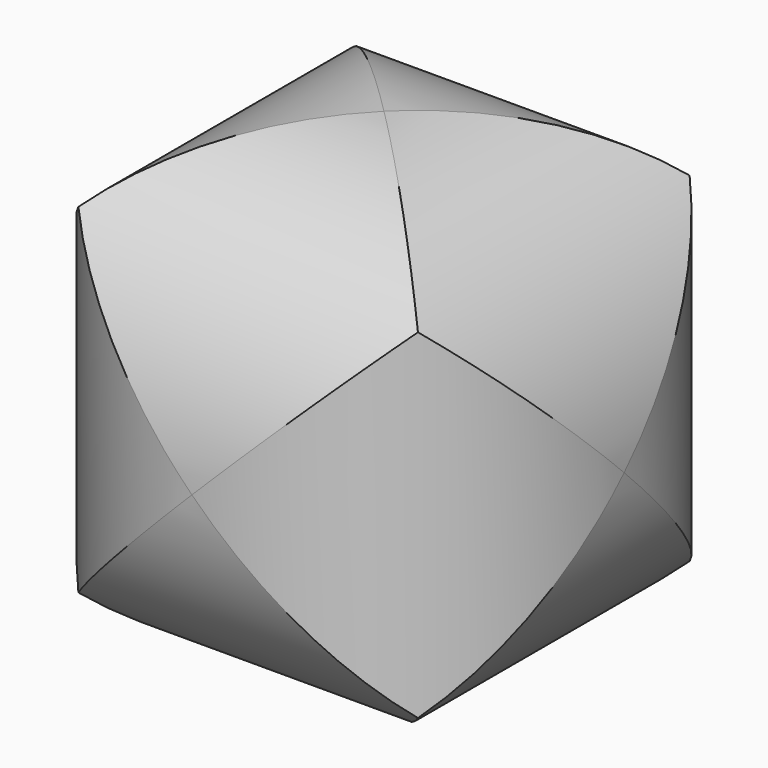
from build123d import *
from build123d import SkipClean  # not in build123d's __all__

# Parameters (mm, degrees)
F0_W     = 76.2
F0_H     = 76.2
F1_DEPTH = 76.2
F5_DEPTH = 76.201
F6_DEPTH = 76.201
F7_DEPTH = 76.201


with BuildPart() as f1:
    # F0 (on Front) → F1 (new body)
    with BuildSketch(Plane.XZ):
        with Locations((38.1, 38.1)):
            Rectangle(F0_W, F0_H)
    extrude(amount=F1_DEPTH)

    # F2 (on face) → F5 (cut, through all)
    with BuildSketch(Plane.XY.offset(76.2)):
        with BuildLine():
            Line((76.2, -76.2), (76.2, -38.1))
            ThreePointArc((76.2, -38.1), (65.0407683632, -65.0407683632), (38.1, -76.2))
            Line((38.1, -76.2), (76.2, -76.2))
        make_face()
        with BuildLine():
            ThreePointArc((38.1, 0), (65.0407683632, -11.1592316368), (76.2, -38.1))
            Line((76.2, -38.1), (76.2, 0))
            Line((76.2, 0), (38.1, 0))
        make_face()
        with BuildLine():
            ThreePointArc((0, -38.1), (11.1592316368, -11.1592316368), (38.1, 0))
            Line((38.1, 0), (0, 0))
            Line((0, 0), (0, -38.1))
        make_face()
        with BuildLine():
            Line((0, -76.2), (38.1, -76.2))
            ThreePointArc((38.1, -76.2), (11.1592316368, -65.0407683632), (0, -38.1))
            Line((0, -38.1), (0, -76.2))
        make_face()
    extrude(amount=-F5_DEPTH, mode=Mode.SUBTRACT)

    # F3 (on face) → F6 (cut, through all)
    with BuildSketch(Plane.XZ.offset(76.2)):
        with BuildLine():
            ThreePointArc((38.1, 76.2), (65.0407683632, 65.0407683632), (76.2, 38.1))
            Line((76.2, 38.1), (76.2, 76.2))
            Line((76.2, 76.2), (38.1, 76.2))
        make_face()
        with BuildLine():
            ThreePointArc((0, 38.1), (11.1592316368, 65.0407683632), (38.1, 76.2))
            Line((38.1, 76.2), (0, 76.2))
            Line((0, 76.2), (0, 38.1))
        make_face()
        with BuildLine():
            Line((76.2, 0), (76.2, 38.1))
            ThreePointArc((76.2, 38.1), (65.0407683632, 11.1592316368), (38.1, 0))
            Line((38.1, 0), (76.2, 0))
        make_face()
        with BuildLine():
            Line((0, 0), (38.1, 0))
            ThreePointArc((38.1, 0), (11.1592316368, 11.1592316368), (0, 38.1))
            Line((0, 38.1), (0, 0))
        make_face()
    extrude(amount=-F6_DEPTH, mode=Mode.SUBTRACT)

    # F4 (on face) → F7 (cut, through all)
    with BuildSketch(Plane.YZ.offset(76.2)):
        with BuildLine():
            ThreePointArc((-38.1, 76.2), (-11.1592316368, 65.0407683632), (0, 38.1))
            Line((0, 38.1), (0, 76.2))
            Line((0, 76.2), (-38.1, 76.2))
        make_face()
        with BuildLine():
            Line((0, 0), (0, 38.1))
            ThreePointArc((0, 38.1), (-11.1592316368, 11.1592316368), (-38.1, 0))
            Line((-38.1, 0), (0, 0))
        make_face()
        with BuildLine():
            Line((-76.2, 0), (-38.1, 0))
            ThreePointArc((-38.1, 0), (-65.0407683632, 11.1592316368), (-76.2, 38.1))
            Line((-76.2, 38.1), (-76.2, 0))
        make_face()
        with BuildLine():
            ThreePointArc((-76.2, 38.1), (-65.0407683632, 65.0407683632), (-38.1, 76.2))
            Line((-38.1, 76.2), (-76.2, 76.2))
            Line((-76.2, 76.2), (-76.2, 38.1))
        make_face()
    with SkipClean():  # cleaning this boolean's faces spoils the solid; the shape is the same uncleaned
        extrude(amount=-F7_DEPTH, mode=Mode.SUBTRACT)


solid = f1.part
